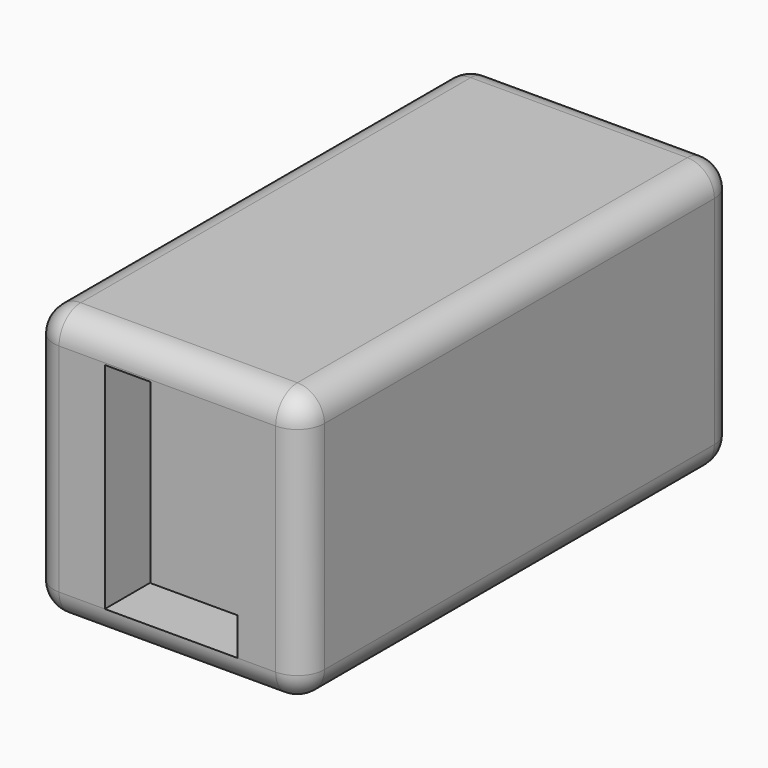
from build123d import *

# Parameters (mm, degrees)
F0_W         = 10
F0_H         = 10
F1_DEPTH     = 20
F2_R         = 1
F3_TEXT_SIZE = 11.1111111111
F4_DEPTH     = 20


# Not quite as in the source:
# - Text() gives the source's letters only with a copy of the font that has no kerning and outlines rounded to 1/6400 em; it was checked with that copy


with BuildPart() as f1:
    # F0 (on Front) → F1 (new body)
    with BuildSketch(Plane.XZ):
        with Locations((5, 5)):
            Rectangle(F0_W, F0_H)
    extrude(amount=F1_DEPTH)

    # F2
    f2_edges = [f1.edges().sort_by_distance(p)[0] for p in [
        (10, -10, 10),
        (0, -10, 10),
        (5, 0, 10),
        (5, -20, 10),
        (10, -10, 0),
        (10, 0, 5),
        (10, -20, 5),
        (0, -10, 0),
        (5, 0, 0),
        (5, -20, 0),
        (0, 0, 5),
        (0, -20, 5),
    ]]
    fillet(f2_edges, radius=F2_R)

    # F3 (on face) → F4 (cut)
    with BuildSketch(Plane.XZ.offset(20)):
        with Locations((1.6909722222, 1)):
            Text('L', F3_TEXT_SIZE, font='Open Sans', font_style=FontStyle.BOLD, text_align=(TextAlign.LEFT, TextAlign.BOTTOM))
    extrude(amount=-F4_DEPTH, mode=Mode.SUBTRACT)


solid = f1.part
